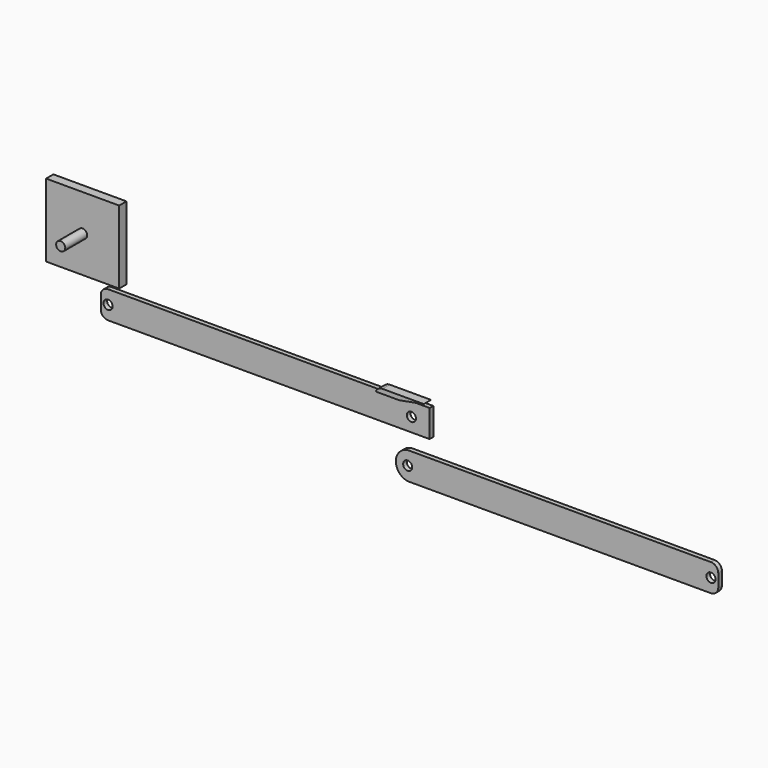
from build123d import *

# Parameters (mm, degrees)
F0_W        = 228.6
F0_H        = 19.05
F0_R        = 3.175
F1_DEPTH    = 3.175
F2_DEPTH    = 3.175
F3_R        = 5.08
F4_R        = 5.08
F5_W        = 34.925
F5_H        = 3.175
F6_DEPTH    = 3.175
F7_T1_DEPTH = 14.9482151929
F7_T3_DEPTH = 14.9482150036
F7_T5_DEPTH = 29.8964301965
F9_DEPTH    = 25.4
F11_DEPTH   = 25.4
F12_R       = 3.175
F13_DEPTH   = 3.176
F14_R       = 3.175
F15_DEPTH   = 6.351
F16_W       = 50.8
F16_H       = 50.8
F16_R       = 3.175
F17_DEPTH   = 6.35
F18_DEPTH   = 25.4


# Not quite as in the source:
# - a fillet or chamfer that OpenCascade refuses, or shapes differently, is made with other operations: its cross-section is extruded or revolved along the edge and cut away or added


with BuildPart() as f1:
    # F0 (on Front) → F1 (new body)
    with BuildSketch(Plane.XZ):
        with Locations((-106.9532044351, 2.9169026516)):
            Rectangle(F0_W, F0_H)
        with Locations((-5.3532044351, 2.9169026516)):
            Circle(F0_R, mode=Mode.SUBTRACT)
    extrude(amount=-F1_DEPTH)

    # F3
    f3_edges = [f1.edges().sort_by_distance(p)[0] for p in [
        (-221.253204, 1.5875, 12.441903),
        (-221.253204, 1.5875, -6.608097),
    ]]
    fillet(f3_edges, radius=F3_R)

    # F5 (on face) → F6 (join)
    with BuildSketch(Plane.XY.offset(12.4419026516)):
        Polygon((10.5217955649, -3.175), (10.5217955649, 3.175), (7.3467955649, 3.175), (7.3467955649, 0), (-27.5782044351, 0), (-27.5782044351, -3.175), align=None)
        with Locations((-10.1157044351, 1.5875)):
            Rectangle(F5_W, F5_H)
    extrude(amount=F6_DEPTH)

    # F7: fillet of radius 5.08 on 2 edges, made by hand

    # F7_s2 → F7_t1 (cut)
    with BuildSketch(Plane.XZ.offset(-14.9482150983)):
        with BuildLine():
            ThreePointArc((-27.5782044351, 12.4419026516), (-25.7087247272, 14.7490161354), (-22.8689183958, 15.6169026516))
            Line((-22.8689183958, 15.6169026516), (-27.5782044351, 15.6169026516))
            Line((-27.5782044351, 15.6169026516), (-27.5782044351, 12.4419026516))
        make_face()
    extrude(amount=F7_T1_DEPTH, mode=Mode.SUBTRACT)

    # F7_s4 → F7_t3 (cut)
    with BuildSketch(Plane.XZ.offset(9.46e-08)):
        with BuildLine():
            ThreePointArc((-27.5782044351, 12.4419026516), (-25.7087247272, 14.7490161354), (-22.8689183958, 15.6169026516))
            Line((-22.8689183958, 15.6169026516), (-27.5782044351, 15.6169026516))
            Line((-27.5782044351, 15.6169026516), (-27.5782044351, 12.4419026516))
        make_face()
    extrude(amount=F7_T3_DEPTH, mode=Mode.SUBTRACT)

    # F7_s6 → F7_t5 (cut)
    with BuildSketch(Plane.XZ.offset(-14.9482150983)):
        with BuildLine():
            ThreePointArc((5.8125095256, 15.6169026516), (8.652315857, 14.7490161354), (10.5217955649, 12.4419026516))
            Line((10.5217955649, 12.4419026516), (10.5217955649, 15.6169026516))
            Line((10.5217955649, 15.6169026516), (5.8125095256, 15.6169026516))
        make_face()
    extrude(amount=F7_T5_DEPTH, mode=Mode.SUBTRACT)

    # F8 (on face) → F9 (cut)
    with BuildSketch(Plane.XZ.offset(3.175)):
        with BuildLine():
            Line((5.8125095256, 15.6169026516), (-11.1592710018, 12.4419026516))
            Line((-11.1592710018, 12.4419026516), (10.5217955649, 12.4419026516))
            ThreePointArc((10.5217955649, 12.4419026516), (8.652315857, 14.7490161354), (5.8125095256, 15.6169026516))
        make_face()
    extrude(amount=-F9_DEPTH, mode=Mode.SUBTRACT)

    # F12 (on face) → F13 (cut, through all)
    with BuildSketch(Plane.XZ):
        with Locations((-216.1732044351, 2.9169026516)):
            Circle(F12_R)
    extrude(amount=-F13_DEPTH, mode=Mode.SUBTRACT)


with BuildPart() as f2:
    # F0 (on Front) → F2 (new body)
    with BuildSketch(Plane.XZ):
        with Locations((96.2467955649, -25.6813844749)):
            Rectangle(F0_W, F0_H)
        with Locations((-5.3532044351, -25.6813844749)):
            Circle(F0_R, mode=Mode.SUBTRACT)
    extrude(amount=F2_DEPTH)

    # F4
    f4_edges = [f2.edges().sort_by_distance(p)[0] for p in [
        (210.546796, -1.5875, -16.156384),
        (210.546796, -1.5875, -35.206384),
    ]]
    fillet(f4_edges, radius=F4_R)

    # F10 (on face) → F11 (cut)
    with BuildSketch(Plane.XZ.offset(3.175)):
        with BuildLine():
            ThreePointArc((-5.3532044351, -35.2063844749), (-13.6081711663, -25.6813844749), (-5.3532044351, -16.1563844749))
            Line((-5.3532044351, -16.1563844749), (-18.0532044351, -16.1563844749))
            Line((-18.0532044351, -16.1563844749), (-18.0532044351, -35.2063844749))
            Line((-18.0532044351, -35.2063844749), (-5.3532044351, -35.2063844749))
        make_face()
    extrude(amount=-F11_DEPTH, mode=Mode.SUBTRACT)

    # F14 (on face) → F15 (cut, through all)
    with BuildSketch(Plane.XZ.offset(3.175)):
        with Locations((205.4667955649, -25.6813844749)):
            Circle(F14_R)
    extrude(amount=-F15_DEPTH, mode=Mode.SUBTRACT)


with BuildPart() as f17:
    # F16 (on Front) → F17 (new body)
    with BuildSketch(Plane.XZ):
        with Locations((-228.7803910017, 44.9747502148)):
            Rectangle(F16_W, F16_H)
        with Locations((-228.7803910017, 44.9747502148)):
            Circle(F16_R, mode=Mode.SUBTRACT)
    extrude(amount=F17_DEPTH)

    # F16 (on Front) → F18 (join)
    with BuildSketch(Plane.XZ):
        with Locations((-228.7803910017, 44.9747502148)):
            Circle(F16_R)
    extrude(amount=F18_DEPTH)


solid = Compound([f1.part, f2.part, f17.part])
